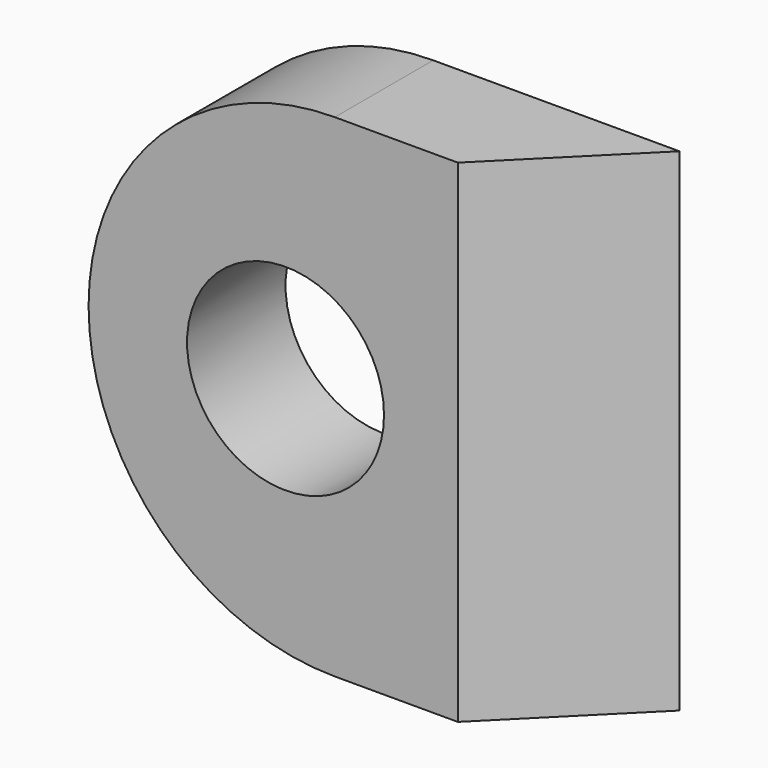
from build123d import *

# Parameters (mm, degrees)
F0_W     = 20
F0_H     = 20
F1_DEPTH = 5
F2_R     = 9.99999
F3_R     = 4
F4_DEPTH = 25
F5_SIZE  = 4.99999


# Not quite as in the source:
# - a fillet or chamfer is up to 0.001 mm smaller than in the source, because OpenCascade refuses the exact size


with BuildPart() as f1:
    # F0 (on Front) → F1 (new body)
    with BuildSketch(Plane.XZ):
        Rectangle(F0_W, F0_H)
    extrude(amount=F1_DEPTH)

    # F2 (radius 10 in the source; OpenCascade refuses exactly that, so slightly less here)
    f2_edges = [f1.edges().sort_by_distance(p)[0] for p in [
        (-10, -2.5, 10),
        (-10, -2.5, -10),
    ]]
    fillet(f2_edges, radius=F2_R)

    # F3 (on face) → F4 (cut)
    with BuildSketch(Plane.XZ.offset(5)):
        with Locations((-2, 0)):
            Circle(F3_R)
    extrude(amount=-F4_DEPTH, mode=Mode.SUBTRACT)

    # F5 (size 5 in the source; OpenCascade refuses exactly that, so slightly less here)
    f5_edges = [f1.edges().sort_by_distance(p)[0] for p in [
        (10, -5, 0),
    ]]
    chamfer(f5_edges, length=F5_SIZE)


solid = f1.part
